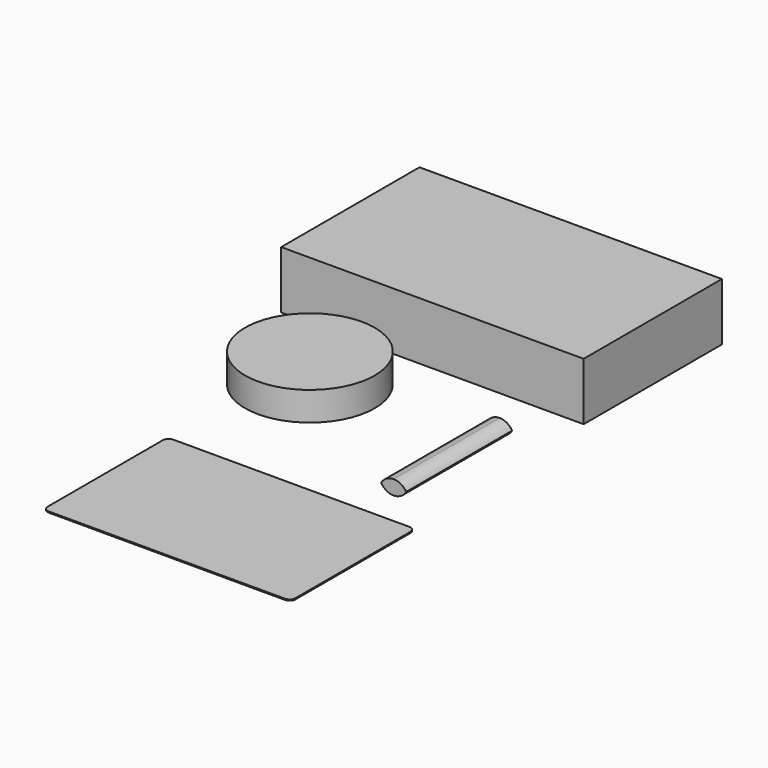
from build123d import *

# Parameters (mm, degrees)
F0_W        = 105
F0_H        = 60
F1_DEPTH    = 20
F2_R        = 22.5
F3_DEPTH    = 10
F5_DEPTH    = 0.4
F6_W        = 10
F6_H        = 46
F7_DEPTH    = 5
F8_T1_DEPTH = 71


# Not quite as in the source:
# - a fillet or chamfer that OpenCascade refuses, or shapes differently, is made with other operations: its cross-section is extruded or revolved along the edge and cut away or added


with BuildPart() as f1:
    # F0 (on Top) → F1 (new body)
    with BuildSketch(Plane.XY):
        with Locations((52.5, 30)):
            Rectangle(F0_W, F0_H)
    extrude(amount=F1_DEPTH)


with BuildPart() as f3:
    # F2 (on Top) → F3 (new body)
    with BuildSketch(Plane.XY):
        with Locations((32.4083268642, -28.0632004142)):
            Circle(F2_R)
    extrude(amount=F3_DEPTH)


with BuildPart() as f5:
    # F4 (on Top) → F5 (new body)
    with BuildSketch(Plane.XY):
        with BuildLine():
            Line((106.2473894497, -77.1431613266), (24.2473894497, -77.1431613266))
            ThreePointArc((24.2473894497, -77.1431613266), (22.8331758874, -77.7289477643), (22.2473894497, -79.1431613266))
            Line((22.2473894497, -79.1431613266), (22.2473894497, -129.1431613266))
            ThreePointArc((22.2473894497, -129.1431613266), (22.8331758874, -130.557374889), (24.2473894497, -131.1431613266))
            Line((24.2473894497, -131.1431613266), (106.2473894497, -131.1431613266))
            ThreePointArc((106.2473894497, -131.1431613266), (107.6616030121, -130.557374889), (108.2473894497, -129.1431613266))
            Line((108.2473894497, -129.1431613266), (108.2473894497, -79.1431613266))
            ThreePointArc((108.2473894497, -79.1431613266), (107.6616030121, -77.7289477643), (106.2473894497, -77.1431613266))
        make_face()
    extrude(amount=F5_DEPTH)


with BuildPart() as f7:
    # F6 (on Top) → F7 (new body)
    with BuildSketch(Plane.XY):
        with Locations((90.8922507425, -41.8344140053)):
            Rectangle(F6_W, F6_H)
    extrude(amount=F7_DEPTH)

    # F8: fillet of radius 5 on 4 edges, made by hand

    # F8_s2 → F8_t1 (cut)
    with BuildSketch(Plane.XZ.offset(6.3344140053)):
        with BuildLine():
            ThreePointArc((95.8922507425, 5), (94.4277846484, 1.4644660941), (90.8922507425, 0))
            Line((90.8922507425, 0), (95.8922507425, 0))
            Line((95.8922507425, 0), (95.8922507425, 5))
        make_face()
        with BuildLine():
            ThreePointArc((85.8922507425, 5), (87.3567168366, 1.4644660941), (90.8922507425, 0))
            Line((90.8922507425, 0), (85.8922507425, 0))
            Line((85.8922507425, 0), (85.8922507425, 5))
        make_face()
        with BuildLine():
            ThreePointArc((85.8922507425, 0), (87.3567168366, 3.5355339059), (90.8922507425, 5))
            Line((90.8922507425, 5), (85.8922507425, 5))
            Line((85.8922507425, 5), (85.8922507425, 0))
        make_face()
        with BuildLine():
            ThreePointArc((95.8922507425, 0), (94.4277846484, 3.5355339059), (90.8922507425, 5))
            Line((90.8922507425, 5), (95.8922507425, 5))
            Line((95.8922507425, 5), (95.8922507425, 0))
        make_face()
    extrude(amount=F8_T1_DEPTH, mode=Mode.SUBTRACT)


solid = Compound([f1.part, f3.part, f5.part, f7.part])
